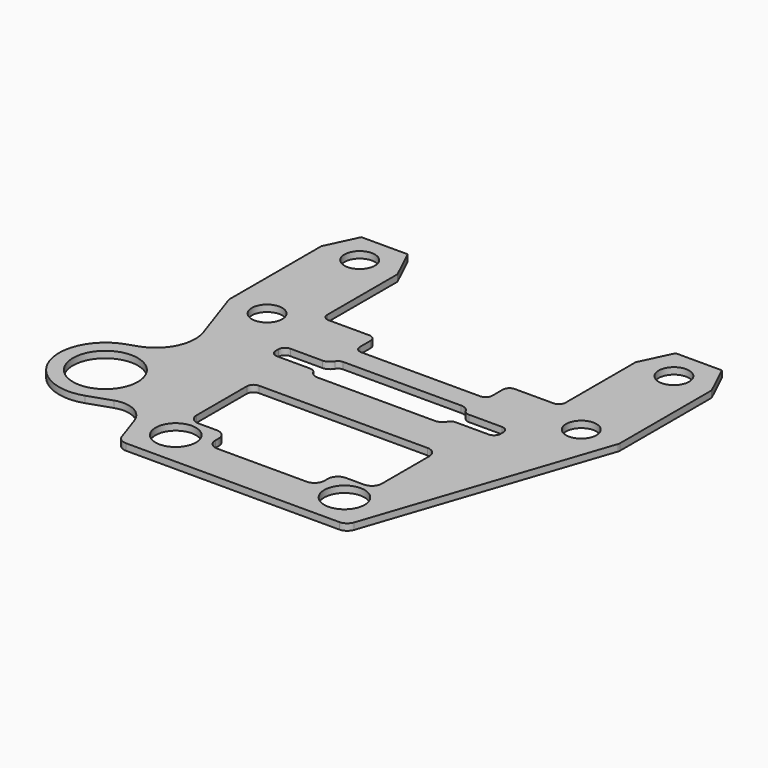
from build123d import *

# Parameters (mm, degrees)
F0_R        = 9.8
F0_R_2      = 6.1
F0_R_3      = 4.6
F1_DEPTH    = 2
F2_R        = 2
F3_R        = 3
F4_W        = 40
F4_H        = 8
F5_DEPTH    = 25
F6_R        = 2
F7_R        = 8
F8_R        = 12
F9_C1_SIZE2 = 4.5
F9_C1_SIZE  = 9.5
F9_C2_SIZE2 = 9.5
F9_C2_SIZE  = 4.5
F9_C3_SIZE2 = 9.5
F9_C3_SIZE  = 4.5
F9_C4_SIZE2 = 9.5
F9_C4_SIZE  = 4.5


# Not quite as in the source:
# - two fillets or chamfers of one size are made in one step


with BuildPart() as f1:
    # F0 (on Top) → F1 (new body)
    with BuildSketch(Plane.XY):
        with BuildLine():
            Line((36, 40.6180607378), (-36, 40.6180607378))
            Line((-36, 40.6180607378), (-36, 78.6180607378))
            Line((-36, 78.6180607378), (-59, 78.6180607378))
            Line((-59, 78.6180607378), (-59, 40.6180607378))
            Line((-59, 40.6180607378), (-59, 34.2180607378))
            Line((-59, 34.2180607378), (-52.466149277, 15.0342559872))
            Line((-52.466149277, 15.0342559872), (-49.3893506198, 6.000577809))
            Line((-49.3893506198, 6.000577809), (-63.7943902368, 1.0943363339))
            ThreePointArc((-63.7943902368, 1.0943363339), (-72.5331453979, -16.6717594171), (-54.7670496468, -25.4105145782))
            Line((-54.7670496468, -25.4105145782), (-40.3620100298, -20.5042731031))
            Line((-40.3620100298, -20.5042731031), (-34.2730196821, -38.3819392622))
            Line((-34.2730196821, -38.3819392622), (34.5899127424, -38.3819392622))
            Line((34.5899127424, -38.3819392622), (59, 34.2180607378))
            Line((59, 34.2180607378), (59, 40.6180607378))
            Line((59, 40.6180607378), (59, 78.6180607378))
            Line((59, 78.6180607378), (36, 78.6180607378))
            Line((36, 78.6180607378), (36, 40.6180607378))
        make_face()
        with Locations((-59.2807199418, -12.1580891221)):
            Circle(F0_R, mode=Mode.SUBTRACT)
        with Locations((-25.5, -27.7819392622)):
            Circle(F0_R_2, mode=Mode.SUBTRACT)
        with Locations((25.5, -27.7819392622)):
            Circle(F0_R_2, mode=Mode.SUBTRACT)
        with BuildLine():
            ThreePointArc((-28, 2.2180607378), (-27.4142135624, 3.6322743002), (-26, 4.2180607378))
            Line((-26, 4.2180607378), (25, 4.2180607378))
            ThreePointArc((25, 4.2180607378), (27.1213203436, 3.3393810814), (28, 1.2180607378))
            Line((28, 1.2180607378), (28, -16.7819392622))
            ThreePointArc((28, -16.7819392622), (27.1213203436, -18.9032596057), (25, -19.7819392622))
            Line((25, -19.7819392622), (19.5, -19.7819392622))
            ThreePointArc((19.5, -19.7819392622), (17.3786796564, -20.6606189186), (16.5, -22.7819392622))
            Line((16.5, -22.7819392622), (16.5, -24.0702618733))
            ThreePointArc((16.5, -24.0702618733), (15.6213203436, -26.1915822169), (13.5, -27.0702618733))
            Line((13.5, -27.0702618733), (-13.5, -27.0702618733))
            ThreePointArc((-13.5, -27.0702618733), (-15.6213203436, -26.1915822169), (-16.5, -24.0702618733))
            Line((-16.5, -24.0702618733), (-16.5, -22.7819392622))
            ThreePointArc((-16.5, -22.7819392622), (-17.3786796564, -20.6606189186), (-19.5, -19.7819392622))
            Line((-19.5, -19.7819392622), (-25, -19.7819392622))
            ThreePointArc((-25, -19.7819392622), (-27.1213203436, -18.9032596057), (-28, -16.7819392622))
            Line((-28, -16.7819392622), (-28, 2.2180607378))
        make_face(mode=Mode.SUBTRACT)
        with Locations((-47.5, 34.2180607378)):
            Circle(F0_R_3, mode=Mode.SUBTRACT)
        with Locations((-47.5, 69.2180607378)):
            Circle(F0_R_3, mode=Mode.SUBTRACT)
        Polygon((-20, 18.6180607378), (-34, 18.6180607378), (-34, 23.6180607378), (-20, 23.6180607378), (-20, 26.1180607378), (20, 26.1180607378), (20, 23.6180607378), (34, 23.6180607378), (34, 18.6180607378), (20, 18.6180607378), (20, 16.1180607378), (-20, 16.1180607378), align=None, mode=Mode.SUBTRACT)
        with Locations((47.5, 34.2180607378)):
            Circle(F0_R_3, mode=Mode.SUBTRACT)
        with Locations((47.5, 69.2180607378)):
            Circle(F0_R_3, mode=Mode.SUBTRACT)
    extrude(amount=F1_DEPTH)

    # F2
    f2_edges = [f1.edges().sort_by_distance(p)[0] for p in [
        (59, 34.218061, 1),
        (-20, 26.118061, 1),
        (20, 23.618061, 1),
        (-34, 23.618061, 1),
        (-20, 18.618061, 1),
        (-34, 18.618061, 1),
        (20, 18.618061, 1),
        (34, 23.618061, 1),
        (34, 18.618061, 1),
        (-59, 34.218061, 1),
        (-36, 40.618061, 1),
        (36, 40.618061, 1),
    ]]
    fillet(f2_edges, radius=F2_R)

    # F3
    f3_edges = [f1.edges().sort_by_distance(p)[0] for p in [
        (-20, 23.618061, 1),
        (-20, 16.118061, 1),
        (20, 26.118061, 1),
        (20, 16.118061, 1),
        (-34.27302, -38.381939, 1),
        (34.589913, -38.381939, 1),
    ]]
    fillet(f3_edges, radius=F3_R)

    # F4 (on face) → F5 (cut)
    with BuildSketch(Plane.XY.offset(2)):
        with Locations((0.2679491924, 36.6180607378)):
            Rectangle(F4_W, F4_H)
    extrude(amount=-F5_DEPTH, mode=Mode.SUBTRACT)

    # F6
    f6_edges = [f1.edges().sort_by_distance(p)[0] for p in [
        (-19.732051, 40.618061, 1),
        (-19.732051, 32.618061, 1),
        (20.267949, 40.618061, 1),
        (20.267949, 32.618061, 1),
    ]]
    fillet(f6_edges, radius=F6_R)

    # F7
    f7_edges = [f1.edges().sort_by_distance(p)[0] for p in [
        (-40.36201, -20.504273, 1),
    ]]
    fillet(f7_edges, radius=F7_R)

    # F8
    f8_edges = [f1.edges().sort_by_distance(p)[0] for p in [
        (-49.389351, 6.000578, 1),
    ]]
    fillet(f8_edges, radius=F8_R)

    # F9: chamfer of 9.5 x 4.5 on 4 edges, made by hand

    # F9_c1
    f9_c1_edges = [f1.edges().sort_by_distance(p)[0] for p in [
        (-59, 78.6180607378, 1),
    ]]
    f9_c1_side = f1.faces().sort_by_distance((-59, 78.5280607378, 1))[0]
    chamfer(f9_c1_edges, length=F9_C1_SIZE, length2=F9_C1_SIZE2, reference=f9_c1_side)

    # F9_c2
    f9_c2_edges = [f1.edges().sort_by_distance(p)[0] for p in [
        (-36, 78.6180607378, 1),
    ]]
    f9_c2_side = f1.faces().sort_by_distance((-36.09, 78.6180607378, 1))[0]
    chamfer(f9_c2_edges, length=F9_C2_SIZE, length2=F9_C2_SIZE2, reference=f9_c2_side)

    # F9_c3
    f9_c3_edges = [f1.edges().sort_by_distance(p)[0] for p in [
        (59, 78.6180607378, 1),
    ]]
    f9_c3_side = f1.faces().sort_by_distance((58.91, 78.6180607378, 1))[0]
    chamfer(f9_c3_edges, length=F9_C3_SIZE, length2=F9_C3_SIZE2, reference=f9_c3_side)

    # F9_c4
    f9_c4_edges = [f1.edges().sort_by_distance(p)[0] for p in [
        (36, 78.6180607378, 1),
    ]]
    f9_c4_side = f1.faces().sort_by_distance((36.09, 78.6180607378, 1))[0]
    chamfer(f9_c4_edges, length=F9_C4_SIZE, length2=F9_C4_SIZE2, reference=f9_c4_side)


solid = f1.part
